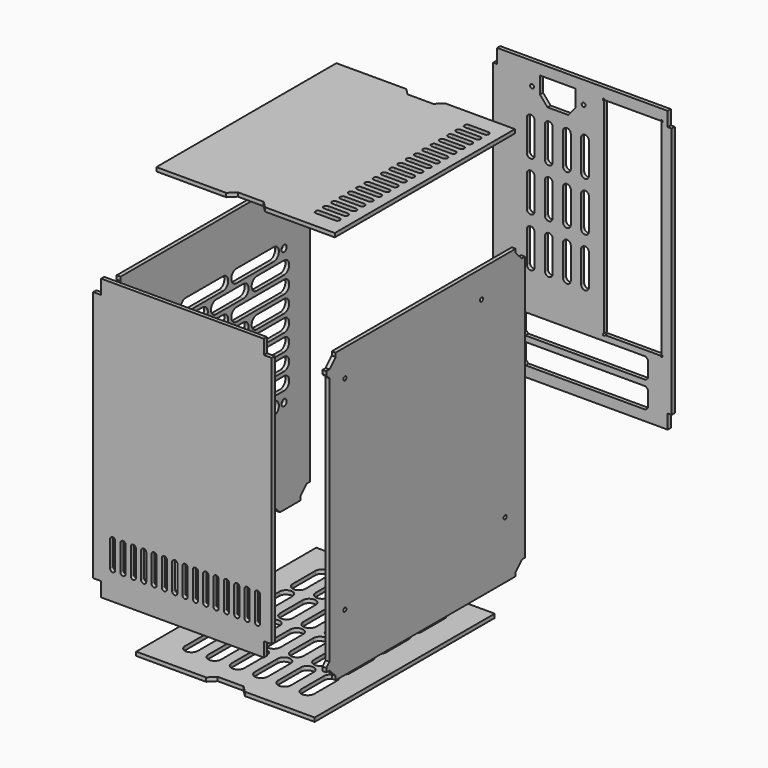
from build123d import *

# Parameters (mm, degrees)
F1_DEPTH  = 3
F4_DEPTH  = 3
F7_DEPTH  = 3
F9_R      = 1.5
F10_DEPTH = 25
F13_DEPTH = 3
F15_R     = 2.5
F16_DEPTH = 25
F19_DEPTH = 3
F22_DEPTH = 25
F25_DEPTH = 3
F29_DEPTH = 25
F31_DEPTH = 3
F33_W     = 97
F33_H     = 15.9
F34_R     = 1.5
F35_DEPTH = 25
F36_SIZE  = 2


# Not quite as in the source:
# - a feature names something its author has since deleted; it is built from what else it names


with BuildPart() as f1:
    # F0 (on Front) → F1 (new body)
    with BuildSketch(Plane.XZ):
        Polygon((53.4554532792, 111.99751333), (-72.3445467208, 111.99751333), (-72.3445467208, 100.89751333), (-78.4445467208, 100.89751333), (-78.4445467208, 3.49751333), (59.5554532792, 3.49751333), (59.5554532792, 100.89751333), (53.4554532792, 100.89751333), align=None)
    extrude(amount=F1_DEPTH)

    # F2: F1 across face


with BuildPart() as f1_1:
    add(f1.part)
    add(f1.part.mirror(Plane(origin=(-9.4445467208, -1.5, 3.49751333), x_dir=(1, 0, 0), z_dir=(0, 0, -1))))

    # F3 (on face) → F4 (cut)
    with BuildSketch(Plane.XZ.offset(3)):
        with BuildLine():
            ThreePointArc((-61.4445467208, -63.00248667), (-63.4445467208, -61.00248667), (-65.4445467208, -63.00248667))
            Line((-65.4445467208, -63.00248667), (-65.4445467208, -83.00248667))
            ThreePointArc((-65.4445467208, -83.00248667), (-63.4445467208, -85.00248667), (-61.4445467208, -83.00248667))
            Line((-61.4445467208, -83.00248667), (-61.4445467208, -63.00248667))
        make_face()
        with BuildLine():
            ThreePointArc((-53.4445467208, -63.00248667), (-55.4445467208, -61.00248667), (-57.4445467208, -63.00248667))
            Line((-57.4445467208, -63.00248667), (-57.4445467208, -83.00248667))
            ThreePointArc((-57.4445467208, -83.00248667), (-55.4445467208, -85.00248667), (-53.4445467208, -83.00248667))
            Line((-53.4445467208, -83.00248667), (-53.4445467208, -63.00248667))
        make_face()
        with BuildLine():
            ThreePointArc((-45.4445467208, -63.00248667), (-47.4445467208, -61.00248667), (-49.4445467208, -63.00248667))
            Line((-49.4445467208, -63.00248667), (-49.4445467208, -83.00248667))
            ThreePointArc((-49.4445467208, -83.00248667), (-47.4445467208, -85.00248667), (-45.4445467208, -83.00248667))
            Line((-45.4445467208, -83.00248667), (-45.4445467208, -63.00248667))
        make_face()
        with BuildLine():
            ThreePointArc((-37.4445467208, -63.00248667), (-39.4445467208, -61.00248667), (-41.4445467208, -63.00248667))
            Line((-41.4445467208, -63.00248667), (-41.4445467208, -83.00248667))
            ThreePointArc((-41.4445467208, -83.00248667), (-39.4445467208, -85.00248667), (-37.4445467208, -83.00248667))
            Line((-37.4445467208, -83.00248667), (-37.4445467208, -63.00248667))
        make_face()
        with BuildLine():
            ThreePointArc((-29.4445467208, -63.00248667), (-31.4445467208, -61.00248667), (-33.4445467208, -63.00248667))
            Line((-33.4445467208, -63.00248667), (-33.4445467208, -83.00248667))
            ThreePointArc((-33.4445467208, -83.00248667), (-31.4445467208, -85.00248667), (-29.4445467208, -83.00248667))
            Line((-29.4445467208, -83.00248667), (-29.4445467208, -63.00248667))
        make_face()
        with BuildLine():
            ThreePointArc((-21.4445467208, -63.00248667), (-23.4445467208, -61.00248667), (-25.4445467208, -63.00248667))
            Line((-25.4445467208, -63.00248667), (-25.4445467208, -83.00248667))
            ThreePointArc((-25.4445467208, -83.00248667), (-23.4445467208, -85.00248667), (-21.4445467208, -83.00248667))
            Line((-21.4445467208, -83.00248667), (-21.4445467208, -63.00248667))
        make_face()
        with BuildLine():
            ThreePointArc((-13.4445467208, -63.00248667), (-15.4445467208, -61.00248667), (-17.4445467208, -63.00248667))
            Line((-17.4445467208, -63.00248667), (-17.4445467208, -83.00248667))
            ThreePointArc((-17.4445467208, -83.00248667), (-15.4445467208, -85.00248667), (-13.4445467208, -83.00248667))
            Line((-13.4445467208, -83.00248667), (-13.4445467208, -63.00248667))
        make_face()
        with BuildLine():
            ThreePointArc((-5.4445467208, -63.00248667), (-7.4445467208, -61.00248667), (-9.4445467208, -63.00248667))
            Line((-9.4445467208, -63.00248667), (-9.4445467208, -83.00248667))
            ThreePointArc((-9.4445467208, -83.00248667), (-7.4445467208, -85.00248667), (-5.4445467208, -83.00248667))
            Line((-5.4445467208, -83.00248667), (-5.4445467208, -63.00248667))
        make_face()
        with BuildLine():
            ThreePointArc((2.5554532792, -63.00248667), (0.5554532792, -61.00248667), (-1.4445467208, -63.00248667))
            Line((-1.4445467208, -63.00248667), (-1.4445467208, -83.00248667))
            ThreePointArc((-1.4445467208, -83.00248667), (0.5554532792, -85.00248667), (2.5554532792, -83.00248667))
            Line((2.5554532792, -83.00248667), (2.5554532792, -63.00248667))
        make_face()
        with BuildLine():
            ThreePointArc((10.5554532792, -63.00248667), (8.5554532792, -61.00248667), (6.5554532792, -63.00248667))
            Line((6.5554532792, -63.00248667), (6.5554532792, -83.00248667))
            ThreePointArc((6.5554532792, -83.00248667), (8.5554532792, -85.00248667), (10.5554532792, -83.00248667))
            Line((10.5554532792, -83.00248667), (10.5554532792, -63.00248667))
        make_face()
        with BuildLine():
            ThreePointArc((18.5554532792, -63.00248667), (16.5554532792, -61.00248667), (14.5554532792, -63.00248667))
            Line((14.5554532792, -63.00248667), (14.5554532792, -83.00248667))
            ThreePointArc((14.5554532792, -83.00248667), (16.5554532792, -85.00248667), (18.5554532792, -83.00248667))
            Line((18.5554532792, -83.00248667), (18.5554532792, -63.00248667))
        make_face()
        with BuildLine():
            ThreePointArc((26.5554532792, -63.00248667), (24.5554532792, -61.00248667), (22.5554532792, -63.00248667))
            Line((22.5554532792, -63.00248667), (22.5554532792, -83.00248667))
            ThreePointArc((22.5554532792, -83.00248667), (24.5554532792, -85.00248667), (26.5554532792, -83.00248667))
            Line((26.5554532792, -83.00248667), (26.5554532792, -63.00248667))
        make_face()
        with BuildLine():
            ThreePointArc((34.5554532792, -63.00248667), (32.5554532792, -61.00248667), (30.5554532792, -63.00248667))
            Line((30.5554532792, -63.00248667), (30.5554532792, -83.00248667))
            ThreePointArc((30.5554532792, -83.00248667), (32.5554532792, -85.00248667), (34.5554532792, -83.00248667))
            Line((34.5554532792, -83.00248667), (34.5554532792, -63.00248667))
        make_face()
        with BuildLine():
            ThreePointArc((42.5554532792, -63.00248667), (40.5554532792, -61.00248667), (38.5554532792, -63.00248667))
            Line((38.5554532792, -63.00248667), (38.5554532792, -83.00248667))
            ThreePointArc((38.5554532792, -83.00248667), (40.5554532792, -85.00248667), (42.5554532792, -83.00248667))
            Line((42.5554532792, -83.00248667), (42.5554532792, -63.00248667))
        make_face()
        with BuildLine():
            ThreePointArc((50.5554532792, -63.00248667), (48.5554532792, -61.00248667), (46.5554532792, -63.00248667))
            Line((46.5554532792, -63.00248667), (46.5554532792, -83.00248667))
            ThreePointArc((46.5554532792, -83.00248667), (48.5554532792, -85.00248667), (50.5554532792, -83.00248667))
            Line((50.5554532792, -83.00248667), (50.5554532792, -63.00248667))
        make_face()
    extrude(amount=-F4_DEPTH, mode=Mode.SUBTRACT)


with BuildPart() as f7:
    # F6 (on offset) → F7 (new body)
    with BuildSketch(Plane.YZ.offset(80)):
        Polygon((203.4780200328, 98.9318754673), (29.4780200328, 98.9318754673), (29.4780200328, 95.9318754673), (23.4780200328, 89.9318754673), (20.4780200328, 89.9318754673), (20.4780200328, 86.9318754673), (23.4780200328, 83.9318754673), (23.4780200328, -12.5681245327), (209.4780200328, -12.5681245327), (209.4780200328, 83.9318754673), (212.4780200328, 86.9318754673), (212.4780200328, 89.9318754673), (209.4780200328, 89.9318754673), (203.4780200328, 95.9318754673), align=None)
        Polygon((212.4780200328, -12.5681245327), (212.4780200328, 86.9318754673), (209.4780200328, 83.9318754673), (209.4780200328, -12.5681245327), align=None)
    extrude(amount=F7_DEPTH)

    # F8: F7 across face


with BuildPart() as f7_1:
    add(f7.part)
    add(f7.part.mirror(Plane(origin=(81.5, 117.9780200328, -12.5681245327), x_dir=(1, 0, 0), z_dir=(0, 0, -1))))

    # F9 (on face) → F10 (cut)
    with BuildSketch(Plane.YZ.offset(83)):
        with Locations((38.3780200328, -79.6681245327)):
            Circle(F9_R)
        with Locations((38.3780200328, 77.7318754673)):
            Circle(F9_R)
        with Locations((170.4780200328, 77.7318754673)):
            Circle(F9_R)
        with Locations((193.2780200328, -79.6681245327)):
            Circle(F9_R)
    extrude(amount=-F10_DEPTH, mode=Mode.SUBTRACT)


with BuildPart() as f13:
    # F12 (on offset) → F13 (new body)
    with BuildSketch(Plane.YZ.offset(-96)):
        Polygon((215.6347262859, 85.4871258276), (215.6347262859, 88.4871258276), (41.6347262859, 88.4871258276), (41.6347262859, 85.4871258276), (35.6347262859, 79.4871258276), (32.6347262859, 79.4871258276), (32.6347262859, 76.4871258276), (35.6347262859, 73.4871258276), (35.6347262859, -23.0128741724), (224.6347262859, -23.0128741724), (224.6347262859, 79.4871258276), (221.6347262859, 79.4871258276), align=None)
    extrude(amount=F13_DEPTH)

    # F14: F13 across face


with BuildPart() as f13_1:
    add(f13.part)
    add(f13.part.mirror(Plane(origin=(-94.5, 130.1347262859, -23.0128741724), x_dir=(1, 0, 0), z_dir=(0, 0, -1))))

    # F15 (on face) → F16 (cut)
    with BuildSketch(Plane(origin=(-96, 0, 0), x_dir=(0, -1, 0), z_dir=(-1, 0, 0))):
        with Locations((-199.6347262859, 43.4871258276)):
            Circle(F15_R)
        with Locations((-94.6347262859, 43.4871258276)):
            Circle(F15_R)
        with BuildLine():
            ThreePointArc((-189.6347262859, 48.4871258276), (-194.6347262859, 43.4871258276), (-189.6347262859, 38.4871258276))
            Line((-189.6347262859, 38.4871258276), (-153.6347262859, 38.4871258276))
            ThreePointArc((-153.6347262859, 38.4871258276), (-148.6347262859, 43.4871258276), (-153.6347262859, 48.4871258276))
            Line((-153.6347262859, 48.4871258276), (-189.6347262859, 48.4871258276))
        make_face()
        with BuildLine():
            ThreePointArc((-140.6347262859, 48.4871258276), (-145.6347262859, 43.4871258276), (-140.6347262859, 38.4871258276))
            Line((-140.6347262859, 38.4871258276), (-104.6347262859, 38.4871258276))
            ThreePointArc((-104.6347262859, 38.4871258276), (-99.6347262859, 43.4871258276), (-104.6347262859, 48.4871258276))
            Line((-104.6347262859, 48.4871258276), (-140.6347262859, 48.4871258276))
        make_face()
        with BuildLine():
            ThreePointArc((-199.6347262859, 35.3621258276), (-204.6347262859, 30.3621258276), (-199.6347262859, 25.3621258276))
            Line((-199.6347262859, 25.3621258276), (-173.3013929526, 25.3621258276))
            ThreePointArc((-173.3013929526, 25.3621258276), (-168.3013929526, 30.3621258276), (-173.3013929526, 35.3621258276))
            Line((-173.3013929526, 35.3621258276), (-199.6347262859, 35.3621258276))
        make_face()
        with BuildLine():
            ThreePointArc((-160.3013929526, 35.3621258276), (-165.3013929526, 30.3621258276), (-160.3013929526, 25.3621258276))
            Line((-160.3013929526, 25.3621258276), (-133.9680596193, 25.3621258276))
            ThreePointArc((-133.9680596193, 25.3621258276), (-128.9680596193, 30.3621258276), (-133.9680596193, 35.3621258276))
            Line((-133.9680596193, 35.3621258276), (-160.3013929526, 35.3621258276))
        make_face()
        with BuildLine():
            ThreePointArc((-120.9680596193, 35.3621258276), (-125.9680596193, 30.3621258276), (-120.9680596193, 25.3621258276))
            Line((-120.9680596193, 25.3621258276), (-94.6347262859, 25.3621258276))
            ThreePointArc((-94.6347262859, 25.3621258276), (-89.6347262859, 30.3621258276), (-94.6347262859, 35.3621258276))
            Line((-94.6347262859, 35.3621258276), (-120.9680596193, 35.3621258276))
        make_face()
        with BuildLine():
            ThreePointArc((-199.6347262859, 22.2371258276), (-204.6347262859, 17.2371258276), (-199.6347262859, 12.2371258276))
            Line((-199.6347262859, 12.2371258276), (-153.6347262859, 12.2371258276))
            ThreePointArc((-153.6347262859, 12.2371258276), (-148.6347262859, 17.2371258276), (-153.6347262859, 22.2371258276))
            Line((-153.6347262859, 22.2371258276), (-199.6347262859, 22.2371258276))
        make_face()
        with BuildLine():
            ThreePointArc((-140.6347262859, 22.2371258276), (-145.6347262859, 17.2371258276), (-140.6347262859, 12.2371258276))
            Line((-140.6347262859, 12.2371258276), (-94.6347262859, 12.2371258276))
            ThreePointArc((-94.6347262859, 12.2371258276), (-89.6347262859, 17.2371258276), (-94.6347262859, 22.2371258276))
            Line((-94.6347262859, 22.2371258276), (-140.6347262859, 22.2371258276))
        make_face()
        with BuildLine():
            ThreePointArc((-199.6347262859, 9.1121258276), (-204.6347262859, 4.1121258276), (-199.6347262859, -0.8878741724))
            Line((-199.6347262859, -0.8878741724), (-173.3013929526, -0.8878741724))
            ThreePointArc((-173.3013929526, -0.8878741724), (-168.3013929526, 4.1121258276), (-173.3013929526, 9.1121258276))
            Line((-173.3013929526, 9.1121258276), (-199.6347262859, 9.1121258276))
        make_face()
        with BuildLine():
            ThreePointArc((-160.3013929526, 9.1121258276), (-165.3013929526, 4.1121258276), (-160.3013929526, -0.8878741724))
            Line((-160.3013929526, -0.8878741724), (-133.9680596193, -0.8878741724))
            ThreePointArc((-133.9680596193, -0.8878741724), (-128.9680596193, 4.1121258276), (-133.9680596193, 9.1121258276))
            Line((-133.9680596193, 9.1121258276), (-160.3013929526, 9.1121258276))
        make_face()
        with BuildLine():
            ThreePointArc((-120.9680596193, 9.1121258276), (-125.9680596193, 4.1121258276), (-120.9680596193, -0.8878741724))
            Line((-120.9680596193, -0.8878741724), (-94.6347262859, -0.8878741724))
            ThreePointArc((-94.6347262859, -0.8878741724), (-89.6347262859, 4.1121258276), (-94.6347262859, 9.1121258276))
            Line((-94.6347262859, 9.1121258276), (-120.9680596193, 9.1121258276))
        make_face()
        with BuildLine():
            ThreePointArc((-199.6347262859, -4.0128741724), (-204.6347262859, -9.0128741724), (-199.6347262859, -14.0128741724))
            Line((-199.6347262859, -14.0128741724), (-153.6347262859, -14.0128741724))
            ThreePointArc((-153.6347262859, -14.0128741724), (-148.6347262859, -9.0128741724), (-153.6347262859, -4.0128741724))
            Line((-153.6347262859, -4.0128741724), (-199.6347262859, -4.0128741724))
        make_face()
        with BuildLine():
            ThreePointArc((-140.6347262859, -4.0128741724), (-145.6347262859, -9.0128741724), (-140.6347262859, -14.0128741724))
            Line((-140.6347262859, -14.0128741724), (-94.6347262859, -14.0128741724))
            ThreePointArc((-94.6347262859, -14.0128741724), (-89.6347262859, -9.0128741724), (-94.6347262859, -4.0128741724))
            Line((-94.6347262859, -4.0128741724), (-140.6347262859, -4.0128741724))
        make_face()
        with BuildLine():
            ThreePointArc((-199.6347262859, -17.1378741724), (-204.6347262859, -22.1378741724), (-199.6347262859, -27.1378741724))
            Line((-199.6347262859, -27.1378741724), (-173.3013929526, -27.1378741724))
            ThreePointArc((-173.3013929526, -27.1378741724), (-168.3013929526, -22.1378741724), (-173.3013929526, -17.1378741724))
            Line((-173.3013929526, -17.1378741724), (-199.6347262859, -17.1378741724))
        make_face()
        with BuildLine():
            ThreePointArc((-160.3013929526, -17.1378741724), (-165.3013929526, -22.1378741724), (-160.3013929526, -27.1378741724))
            Line((-160.3013929526, -27.1378741724), (-133.9680596193, -27.1378741724))
            ThreePointArc((-133.9680596193, -27.1378741724), (-128.9680596193, -22.1378741724), (-133.9680596193, -17.1378741724))
            Line((-133.9680596193, -17.1378741724), (-160.3013929526, -17.1378741724))
        make_face()
        with BuildLine():
            ThreePointArc((-120.9680596193, -17.1378741724), (-125.9680596193, -22.1378741724), (-120.9680596193, -27.1378741724))
            Line((-120.9680596193, -27.1378741724), (-94.6347262859, -27.1378741724))
            ThreePointArc((-94.6347262859, -27.1378741724), (-89.6347262859, -22.1378741724), (-94.6347262859, -17.1378741724))
            Line((-94.6347262859, -17.1378741724), (-120.9680596193, -17.1378741724))
        make_face()
        with BuildLine():
            ThreePointArc((-199.6347262859, -30.2628741724), (-204.6347262859, -35.2628741724), (-199.6347262859, -40.2628741724))
            Line((-199.6347262859, -40.2628741724), (-153.6347262859, -40.2628741724))
            ThreePointArc((-153.6347262859, -40.2628741724), (-148.6347262859, -35.2628741724), (-153.6347262859, -30.2628741724))
            Line((-153.6347262859, -30.2628741724), (-199.6347262859, -30.2628741724))
        make_face()
        with BuildLine():
            ThreePointArc((-140.6347262859, -30.2628741724), (-145.6347262859, -35.2628741724), (-140.6347262859, -40.2628741724))
            Line((-140.6347262859, -40.2628741724), (-94.6347262859, -40.2628741724))
            ThreePointArc((-94.6347262859, -40.2628741724), (-89.6347262859, -35.2628741724), (-94.6347262859, -30.2628741724))
            Line((-94.6347262859, -30.2628741724), (-140.6347262859, -30.2628741724))
        make_face()
        with BuildLine():
            ThreePointArc((-199.6347262859, -43.3878741724), (-204.6347262859, -48.3878741724), (-199.6347262859, -53.3878741724))
            Line((-199.6347262859, -53.3878741724), (-173.3013929526, -53.3878741724))
            ThreePointArc((-173.3013929526, -53.3878741724), (-168.3013929526, -48.3878741724), (-173.3013929526, -43.3878741724))
            Line((-173.3013929526, -43.3878741724), (-199.6347262859, -43.3878741724))
        make_face()
        with BuildLine():
            ThreePointArc((-160.3013929526, -43.3878741724), (-165.3013929526, -48.3878741724), (-160.3013929526, -53.3878741724))
            Line((-160.3013929526, -53.3878741724), (-133.9680596193, -53.3878741724))
            ThreePointArc((-133.9680596193, -53.3878741724), (-128.9680596193, -48.3878741724), (-133.9680596193, -43.3878741724))
            Line((-133.9680596193, -43.3878741724), (-160.3013929526, -43.3878741724))
        make_face()
        with BuildLine():
            ThreePointArc((-120.9680596193, -43.3878741724), (-125.9680596193, -48.3878741724), (-120.9680596193, -53.3878741724))
            Line((-120.9680596193, -53.3878741724), (-94.6347262859, -53.3878741724))
            ThreePointArc((-94.6347262859, -53.3878741724), (-89.6347262859, -48.3878741724), (-94.6347262859, -43.3878741724))
            Line((-94.6347262859, -43.3878741724), (-120.9680596193, -43.3878741724))
        make_face()
        with BuildLine():
            ThreePointArc((-189.6347262859, -56.5128741724), (-194.6347262859, -61.5128741724), (-189.6347262859, -66.5128741724))
            Line((-189.6347262859, -66.5128741724), (-153.6347262859, -66.5128741724))
            ThreePointArc((-153.6347262859, -66.5128741724), (-148.6347262859, -61.5128741724), (-153.6347262859, -56.5128741724))
            Line((-153.6347262859, -56.5128741724), (-189.6347262859, -56.5128741724))
        make_face()
        with BuildLine():
            ThreePointArc((-140.6347262859, -56.5128741724), (-145.6347262859, -61.5128741724), (-140.6347262859, -66.5128741724))
            Line((-140.6347262859, -66.5128741724), (-104.6347262859, -66.5128741724))
            ThreePointArc((-104.6347262859, -66.5128741724), (-99.6347262859, -61.5128741724), (-104.6347262859, -56.5128741724))
            Line((-104.6347262859, -56.5128741724), (-140.6347262859, -56.5128741724))
        make_face()
        with Locations((-199.6347262859, -61.5128741724)):
            Circle(F15_R)
        with Locations((-94.6347262859, -61.5128741724)):
            Circle(F15_R)
        Polygon((-187.6347262859, -126.5128741724), (-195.6347262859, -134.5128741724), (-61.6347262859, -134.5128741724), (-69.6347262859, -126.5128741724), align=None)
    extrude(amount=-F16_DEPTH, mode=Mode.SUBTRACT)


with BuildPart() as f19:
    # F18 (on offset) → F19 (new body)
    with BuildSketch(Plane.XY.offset(155)):
        Polygon((55.7591726665, 149.7526661158), (-82.2408273335, 149.7526661158), (-82.2408273335, 62.7526661158), (-28.2408273335, 62.7526661158), (-23.2408273335, 67.7526661158), (-13.2408273335, 67.7526661158), (-3.2408273335, 67.7526661158), (1.7591726665, 62.7526661158), (55.7591726665, 62.7526661158), align=None)
    extrude(amount=F19_DEPTH)

    # F20: F19 across face


with BuildPart() as f19_1:
    add(f19.part)
    add(f19.part.mirror(Plane(origin=(-13.2408273335, 149.7526661158, 156.5), x_dir=(-1, 0, 0), z_dir=(0, 1, 0))))

    # F21 (on face) → F22 (cut)
    with BuildSketch(Plane.XY.offset(158)):
        with BuildLine():
            ThreePointArc((30.7591726665, 79.7526661158), (28.7591726665, 77.7526661158), (30.7591726665, 75.7526661158))
            Line((30.7591726665, 75.7526661158), (45.7591726665, 75.7526661158))
            ThreePointArc((45.7591726665, 75.7526661158), (47.7591726665, 77.7526661158), (45.7591726665, 79.7526661158))
            Line((45.7591726665, 79.7526661158), (30.7591726665, 79.7526661158))
        make_face()
        with BuildLine():
            ThreePointArc((30.7591726665, 87.7526661158), (28.7591726665, 85.7526661158), (30.7591726665, 83.7526661158))
            Line((30.7591726665, 83.7526661158), (45.7591726665, 83.7526661158))
            ThreePointArc((45.7591726665, 83.7526661158), (47.7591726665, 85.7526661158), (45.7591726665, 87.7526661158))
            Line((45.7591726665, 87.7526661158), (30.7591726665, 87.7526661158))
        make_face()
        with BuildLine():
            ThreePointArc((30.7591726665, 95.7526661158), (28.7591726665, 93.7526661158), (30.7591726665, 91.7526661158))
            Line((30.7591726665, 91.7526661158), (45.7591726665, 91.7526661158))
            ThreePointArc((45.7591726665, 91.7526661158), (47.7591726665, 93.7526661158), (45.7591726665, 95.7526661158))
            Line((45.7591726665, 95.7526661158), (30.7591726665, 95.7526661158))
        make_face()
        with BuildLine():
            ThreePointArc((30.7591726665, 103.7526661158), (28.7591726665, 101.7526661158), (30.7591726665, 99.7526661158))
            Line((30.7591726665, 99.7526661158), (45.7591726665, 99.7526661158))
            ThreePointArc((45.7591726665, 99.7526661158), (47.7591726665, 101.7526661158), (45.7591726665, 103.7526661158))
            Line((45.7591726665, 103.7526661158), (30.7591726665, 103.7526661158))
        make_face()
        with BuildLine():
            ThreePointArc((30.7591726665, 111.7526661158), (28.7591726665, 109.7526661158), (30.7591726665, 107.7526661158))
            Line((30.7591726665, 107.7526661158), (45.7591726665, 107.7526661158))
            ThreePointArc((45.7591726665, 107.7526661158), (47.7591726665, 109.7526661158), (45.7591726665, 111.7526661158))
            Line((45.7591726665, 111.7526661158), (30.7591726665, 111.7526661158))
        make_face()
        with BuildLine():
            ThreePointArc((30.7591726665, 119.7526661158), (28.7591726665, 117.7526661158), (30.7591726665, 115.7526661158))
            Line((30.7591726665, 115.7526661158), (45.7591726665, 115.7526661158))
            ThreePointArc((45.7591726665, 115.7526661158), (47.7591726665, 117.7526661158), (45.7591726665, 119.7526661158))
            Line((45.7591726665, 119.7526661158), (30.7591726665, 119.7526661158))
        make_face()
        with BuildLine():
            ThreePointArc((30.7591726665, 127.7526661158), (28.7591726665, 125.7526661158), (30.7591726665, 123.7526661158))
            Line((30.7591726665, 123.7526661158), (45.7591726665, 123.7526661158))
            ThreePointArc((45.7591726665, 123.7526661158), (47.7591726665, 125.7526661158), (45.7591726665, 127.7526661158))
            Line((45.7591726665, 127.7526661158), (30.7591726665, 127.7526661158))
        make_face()
        with BuildLine():
            ThreePointArc((30.7591726665, 135.7526661158), (28.7591726665, 133.7526661158), (30.7591726665, 131.7526661158))
            Line((30.7591726665, 131.7526661158), (45.7591726665, 131.7526661158))
            ThreePointArc((45.7591726665, 131.7526661158), (47.7591726665, 133.7526661158), (45.7591726665, 135.7526661158))
            Line((45.7591726665, 135.7526661158), (30.7591726665, 135.7526661158))
        make_face()
        with BuildLine():
            ThreePointArc((30.7591726665, 143.7526661158), (28.7591726665, 141.7526661158), (30.7591726665, 139.7526661158))
            Line((30.7591726665, 139.7526661158), (45.7591726665, 139.7526661158))
            ThreePointArc((45.7591726665, 139.7526661158), (47.7591726665, 141.7526661158), (45.7591726665, 143.7526661158))
            Line((45.7591726665, 143.7526661158), (30.7591726665, 143.7526661158))
        make_face()
        with BuildLine():
            ThreePointArc((30.7591726665, 151.7526661158), (28.7591726665, 149.7526661158), (30.7591726665, 147.7526661158))
            Line((30.7591726665, 147.7526661158), (45.7591726665, 147.7526661158))
            ThreePointArc((45.7591726665, 147.7526661158), (47.7591726665, 149.7526661158), (45.7591726665, 151.7526661158))
            Line((45.7591726665, 151.7526661158), (30.7591726665, 151.7526661158))
        make_face()
        with BuildLine():
            ThreePointArc((30.7591726665, 159.7526661158), (28.7591726665, 157.7526661158), (30.7591726665, 155.7526661158))
            Line((30.7591726665, 155.7526661158), (45.7591726665, 155.7526661158))
            ThreePointArc((45.7591726665, 155.7526661158), (47.7591726665, 157.7526661158), (45.7591726665, 159.7526661158))
            Line((45.7591726665, 159.7526661158), (30.7591726665, 159.7526661158))
        make_face()
        with BuildLine():
            ThreePointArc((30.7591726665, 167.7526661158), (28.7591726665, 165.7526661158), (30.7591726665, 163.7526661158))
            Line((30.7591726665, 163.7526661158), (45.7591726665, 163.7526661158))
            ThreePointArc((45.7591726665, 163.7526661158), (47.7591726665, 165.7526661158), (45.7591726665, 167.7526661158))
            Line((45.7591726665, 167.7526661158), (30.7591726665, 167.7526661158))
        make_face()
        with BuildLine():
            ThreePointArc((30.7591726665, 175.7526661158), (28.7591726665, 173.7526661158), (30.7591726665, 171.7526661158))
            Line((30.7591726665, 171.7526661158), (45.7591726665, 171.7526661158))
            ThreePointArc((45.7591726665, 171.7526661158), (47.7591726665, 173.7526661158), (45.7591726665, 175.7526661158))
            Line((45.7591726665, 175.7526661158), (30.7591726665, 175.7526661158))
        make_face()
        with BuildLine():
            ThreePointArc((30.7591726665, 183.7526661158), (28.7591726665, 181.7526661158), (30.7591726665, 179.7526661158))
            Line((30.7591726665, 179.7526661158), (45.7591726665, 179.7526661158))
            ThreePointArc((45.7591726665, 179.7526661158), (47.7591726665, 181.7526661158), (45.7591726665, 183.7526661158))
            Line((45.7591726665, 183.7526661158), (30.7591726665, 183.7526661158))
        make_face()
        with BuildLine():
            ThreePointArc((30.7591726665, 191.7526661158), (28.7591726665, 189.7526661158), (30.7591726665, 187.7526661158))
            Line((30.7591726665, 187.7526661158), (45.7591726665, 187.7526661158))
            ThreePointArc((45.7591726665, 187.7526661158), (47.7591726665, 189.7526661158), (45.7591726665, 191.7526661158))
            Line((45.7591726665, 191.7526661158), (30.7591726665, 191.7526661158))
        make_face()
        with BuildLine():
            ThreePointArc((30.7591726665, 199.7526661158), (28.7591726665, 197.7526661158), (30.7591726665, 195.7526661158))
            Line((30.7591726665, 195.7526661158), (45.7591726665, 195.7526661158))
            ThreePointArc((45.7591726665, 195.7526661158), (47.7591726665, 197.7526661158), (45.7591726665, 199.7526661158))
            Line((45.7591726665, 199.7526661158), (30.7591726665, 199.7526661158))
        make_face()
        with BuildLine():
            ThreePointArc((30.7591726665, 207.7526661158), (28.7591726665, 205.7526661158), (30.7591726665, 203.7526661158))
            Line((30.7591726665, 203.7526661158), (45.7591726665, 203.7526661158))
            ThreePointArc((45.7591726665, 203.7526661158), (47.7591726665, 205.7526661158), (45.7591726665, 207.7526661158))
            Line((45.7591726665, 207.7526661158), (30.7591726665, 207.7526661158))
        make_face()
        with BuildLine():
            ThreePointArc((30.7591726665, 215.7526661158), (28.7591726665, 213.7526661158), (30.7591726665, 211.7526661158))
            Line((30.7591726665, 211.7526661158), (45.7591726665, 211.7526661158))
            ThreePointArc((45.7591726665, 211.7526661158), (47.7591726665, 213.7526661158), (45.7591726665, 215.7526661158))
            Line((45.7591726665, 215.7526661158), (30.7591726665, 215.7526661158))
        make_face()
        with BuildLine():
            ThreePointArc((30.7591726665, 223.7526661158), (28.7591726665, 221.7526661158), (30.7591726665, 219.7526661158))
            Line((30.7591726665, 219.7526661158), (45.7591726665, 219.7526661158))
            ThreePointArc((45.7591726665, 219.7526661158), (47.7591726665, 221.7526661158), (45.7591726665, 223.7526661158))
            Line((45.7591726665, 223.7526661158), (30.7591726665, 223.7526661158))
        make_face()
    extrude(amount=-F22_DEPTH, mode=Mode.SUBTRACT)


with BuildPart() as f25:
    # F24 (on offset) → F25 (new body)
    with BuildSketch(Plane.XY.offset(-153)):
        Polygon((-65.5607343912, 109.4242391139), (-65.5607343912, 22.4242391139), (-11.5607343912, 22.4242391139), (-6.5607343912, 27.4242391139), (3.4392656088, 27.4242391139), (13.4392656088, 27.4242391139), (18.4392656088, 22.4242391139), (72.4392656088, 22.4242391139), (72.4392656088, 109.4242391139), align=None)
    extrude(amount=F25_DEPTH)

    # F26: F25 across face


with BuildPart() as f25_1:
    add(f25.part)
    add(f25.part.mirror(Plane(origin=(3.4392656088, 109.4242391139, -151.5), x_dir=(-1, 0, 0), z_dir=(0, 1, 0))))

    # F28 (on face) → F29 (cut)
    with BuildSketch(Plane(origin=(0, 0, -153), x_dir=(1, 0, 0), z_dir=(0, 0, -1))):
        with BuildLine():
            ThreePointArc((-47.0607343912, -172.4242391139), (-42.0607343912, -177.4242391139), (-37.0607343912, -172.4242391139))
            Line((-37.0607343912, -172.4242391139), (-37.0607343912, -150.4242391139))
            ThreePointArc((-37.0607343912, -150.4242391139), (-42.0607343912, -145.4242391139), (-47.0607343912, -150.4242391139))
            Line((-47.0607343912, -150.4242391139), (-47.0607343912, -172.4242391139))
        make_face()
        with BuildLine():
            ThreePointArc((-47.0607343912, -137.7575724473), (-42.0607343912, -142.7575724473), (-37.0607343912, -137.7575724473))
            Line((-37.0607343912, -137.7575724473), (-37.0607343912, -115.7575724473))
            ThreePointArc((-37.0607343912, -115.7575724473), (-42.0607343912, -110.7575724473), (-47.0607343912, -115.7575724473))
            Line((-47.0607343912, -115.7575724473), (-47.0607343912, -137.7575724473))
        make_face()
        with BuildLine():
            ThreePointArc((-47.0607343912, -103.0909057806), (-42.0607343912, -108.0909057806), (-37.0607343912, -103.0909057806))
            Line((-37.0607343912, -103.0909057806), (-37.0607343912, -81.0909057806))
            ThreePointArc((-37.0607343912, -81.0909057806), (-42.0607343912, -76.0909057806), (-47.0607343912, -81.0909057806))
            Line((-47.0607343912, -81.0909057806), (-47.0607343912, -103.0909057806))
        make_face()
        with BuildLine():
            ThreePointArc((-47.0607343912, -68.4242391139), (-42.0607343912, -73.4242391139), (-37.0607343912, -68.4242391139))
            Line((-37.0607343912, -68.4242391139), (-37.0607343912, -46.4242391139))
            ThreePointArc((-37.0607343912, -46.4242391139), (-42.0607343912, -41.4242391139), (-47.0607343912, -46.4242391139))
            Line((-47.0607343912, -46.4242391139), (-47.0607343912, -68.4242391139))
        make_face()
        with BuildLine():
            ThreePointArc((-29.0607343912, -172.4242391139), (-24.0607343912, -177.4242391139), (-19.0607343912, -172.4242391139))
            Line((-19.0607343912, -172.4242391139), (-19.0607343912, -150.4242391139))
            ThreePointArc((-19.0607343912, -150.4242391139), (-24.0607343912, -145.4242391139), (-29.0607343912, -150.4242391139))
            Line((-29.0607343912, -150.4242391139), (-29.0607343912, -172.4242391139))
        make_face()
        with BuildLine():
            ThreePointArc((-29.0607343912, -137.7575724473), (-24.0607343912, -142.7575724473), (-19.0607343912, -137.7575724473))
            Line((-19.0607343912, -137.7575724473), (-19.0607343912, -115.7575724473))
            ThreePointArc((-19.0607343912, -115.7575724473), (-24.0607343912, -110.7575724473), (-29.0607343912, -115.7575724473))
            Line((-29.0607343912, -115.7575724473), (-29.0607343912, -137.7575724473))
        make_face()
        with BuildLine():
            ThreePointArc((-29.0607343912, -103.0909057806), (-24.0607343912, -108.0909057806), (-19.0607343912, -103.0909057806))
            Line((-19.0607343912, -103.0909057806), (-19.0607343912, -81.0909057806))
            ThreePointArc((-19.0607343912, -81.0909057806), (-24.0607343912, -76.0909057806), (-29.0607343912, -81.0909057806))
            Line((-29.0607343912, -81.0909057806), (-29.0607343912, -103.0909057806))
        make_face()
        with BuildLine():
            ThreePointArc((-29.0607343912, -68.4242391139), (-24.0607343912, -73.4242391139), (-19.0607343912, -68.4242391139))
            Line((-19.0607343912, -68.4242391139), (-19.0607343912, -46.4242391139))
            ThreePointArc((-19.0607343912, -46.4242391139), (-24.0607343912, -41.4242391139), (-29.0607343912, -46.4242391139))
            Line((-29.0607343912, -46.4242391139), (-29.0607343912, -68.4242391139))
        make_face()
        with BuildLine():
            ThreePointArc((-11.0607343912, -172.4242391139), (-6.0607343912, -177.4242391139), (-1.0607343912, -172.4242391139))
            Line((-1.0607343912, -172.4242391139), (-1.0607343912, -150.4242391139))
            ThreePointArc((-1.0607343912, -150.4242391139), (-6.0607343912, -145.4242391139), (-11.0607343912, -150.4242391139))
            Line((-11.0607343912, -150.4242391139), (-11.0607343912, -172.4242391139))
        make_face()
        with BuildLine():
            ThreePointArc((-11.0607343912, -137.7575724473), (-6.0607343912, -142.7575724473), (-1.0607343912, -137.7575724473))
            Line((-1.0607343912, -137.7575724473), (-1.0607343912, -115.7575724473))
            ThreePointArc((-1.0607343912, -115.7575724473), (-6.0607343912, -110.7575724473), (-11.0607343912, -115.7575724473))
            Line((-11.0607343912, -115.7575724473), (-11.0607343912, -137.7575724473))
        make_face()
        with BuildLine():
            ThreePointArc((-11.0607343912, -103.0909057806), (-6.0607343912, -108.0909057806), (-1.0607343912, -103.0909057806))
            Line((-1.0607343912, -103.0909057806), (-1.0607343912, -81.0909057806))
            ThreePointArc((-1.0607343912, -81.0909057806), (-6.0607343912, -76.0909057806), (-11.0607343912, -81.0909057806))
            Line((-11.0607343912, -81.0909057806), (-11.0607343912, -103.0909057806))
        make_face()
        with BuildLine():
            ThreePointArc((-11.0607343912, -68.4242391139), (-6.0607343912, -73.4242391139), (-1.0607343912, -68.4242391139))
            Line((-1.0607343912, -68.4242391139), (-1.0607343912, -46.4242391139))
            ThreePointArc((-1.0607343912, -46.4242391139), (-6.0607343912, -41.4242391139), (-11.0607343912, -46.4242391139))
            Line((-11.0607343912, -46.4242391139), (-11.0607343912, -68.4242391139))
        make_face()
        with BuildLine():
            ThreePointArc((6.9392656088, -172.4242391139), (11.9392656088, -177.4242391139), (16.9392656088, -172.4242391139))
            Line((16.9392656088, -172.4242391139), (16.9392656088, -150.4242391139))
            ThreePointArc((16.9392656088, -150.4242391139), (11.9392656088, -145.4242391139), (6.9392656088, -150.4242391139))
            Line((6.9392656088, -150.4242391139), (6.9392656088, -172.4242391139))
        make_face()
        with BuildLine():
            ThreePointArc((6.9392656088, -137.7575724473), (11.9392656088, -142.7575724473), (16.9392656088, -137.7575724473))
            Line((16.9392656088, -137.7575724473), (16.9392656088, -115.7575724473))
            ThreePointArc((16.9392656088, -115.7575724473), (11.9392656088, -110.7575724473), (6.9392656088, -115.7575724473))
            Line((6.9392656088, -115.7575724473), (6.9392656088, -137.7575724473))
        make_face()
        with BuildLine():
            ThreePointArc((6.9392656088, -103.0909057806), (11.9392656088, -108.0909057806), (16.9392656088, -103.0909057806))
            Line((16.9392656088, -103.0909057806), (16.9392656088, -81.0909057806))
            ThreePointArc((16.9392656088, -81.0909057806), (11.9392656088, -76.0909057806), (6.9392656088, -81.0909057806))
            Line((6.9392656088, -81.0909057806), (6.9392656088, -103.0909057806))
        make_face()
        with BuildLine():
            ThreePointArc((6.9392656088, -68.4242391139), (11.9392656088, -73.4242391139), (16.9392656088, -68.4242391139))
            Line((16.9392656088, -68.4242391139), (16.9392656088, -46.4242391139))
            ThreePointArc((16.9392656088, -46.4242391139), (11.9392656088, -41.4242391139), (6.9392656088, -46.4242391139))
            Line((6.9392656088, -46.4242391139), (6.9392656088, -68.4242391139))
        make_face()
        with BuildLine():
            ThreePointArc((24.9392656088, -172.4242391139), (29.9392656088, -177.4242391139), (34.9392656088, -172.4242391139))
            Line((34.9392656088, -172.4242391139), (34.9392656088, -150.4242391139))
            ThreePointArc((34.9392656088, -150.4242391139), (29.9392656088, -145.4242391139), (24.9392656088, -150.4242391139))
            Line((24.9392656088, -150.4242391139), (24.9392656088, -172.4242391139))
        make_face()
        with BuildLine():
            ThreePointArc((24.9392656088, -137.7575724473), (29.9392656088, -142.7575724473), (34.9392656088, -137.7575724473))
            Line((34.9392656088, -137.7575724473), (34.9392656088, -115.7575724473))
            ThreePointArc((34.9392656088, -115.7575724473), (29.9392656088, -110.7575724473), (24.9392656088, -115.7575724473))
            Line((24.9392656088, -115.7575724473), (24.9392656088, -137.7575724473))
        make_face()
        with BuildLine():
            ThreePointArc((24.9392656088, -103.0909057806), (29.9392656088, -108.0909057806), (34.9392656088, -103.0909057806))
            Line((34.9392656088, -103.0909057806), (34.9392656088, -81.0909057806))
            ThreePointArc((34.9392656088, -81.0909057806), (29.9392656088, -76.0909057806), (24.9392656088, -81.0909057806))
            Line((24.9392656088, -81.0909057806), (24.9392656088, -103.0909057806))
        make_face()
        with BuildLine():
            ThreePointArc((24.9392656088, -68.4242391139), (29.9392656088, -73.4242391139), (34.9392656088, -68.4242391139))
            Line((34.9392656088, -68.4242391139), (34.9392656088, -46.4242391139))
            ThreePointArc((34.9392656088, -46.4242391139), (29.9392656088, -41.4242391139), (24.9392656088, -46.4242391139))
            Line((24.9392656088, -46.4242391139), (24.9392656088, -68.4242391139))
        make_face()
        with BuildLine():
            ThreePointArc((42.9392656088, -172.4242391139), (47.9392656088, -177.4242391139), (52.9392656088, -172.4242391139))
            Line((52.9392656088, -172.4242391139), (52.9392656088, -150.4242391139))
            ThreePointArc((52.9392656088, -150.4242391139), (47.9392656088, -145.4242391139), (42.9392656088, -150.4242391139))
            Line((42.9392656088, -150.4242391139), (42.9392656088, -172.4242391139))
        make_face()
        with BuildLine():
            ThreePointArc((42.9392656088, -137.7575724473), (47.9392656088, -142.7575724473), (52.9392656088, -137.7575724473))
            Line((52.9392656088, -137.7575724473), (52.9392656088, -115.7575724473))
            ThreePointArc((52.9392656088, -115.7575724473), (47.9392656088, -110.7575724473), (42.9392656088, -115.7575724473))
            Line((42.9392656088, -115.7575724473), (42.9392656088, -137.7575724473))
        make_face()
        with BuildLine():
            ThreePointArc((42.9392656088, -103.0909057806), (47.9392656088, -108.0909057806), (52.9392656088, -103.0909057806))
            Line((52.9392656088, -103.0909057806), (52.9392656088, -81.0909057806))
            ThreePointArc((52.9392656088, -81.0909057806), (47.9392656088, -76.0909057806), (42.9392656088, -81.0909057806))
            Line((42.9392656088, -81.0909057806), (42.9392656088, -103.0909057806))
        make_face()
        with BuildLine():
            ThreePointArc((42.9392656088, -68.4242391139), (47.9392656088, -73.4242391139), (52.9392656088, -68.4242391139))
            Line((52.9392656088, -68.4242391139), (52.9392656088, -46.4242391139))
            ThreePointArc((52.9392656088, -46.4242391139), (47.9392656088, -41.4242391139), (42.9392656088, -46.4242391139))
            Line((42.9392656088, -46.4242391139), (42.9392656088, -68.4242391139))
        make_face()
    extrude(amount=-F29_DEPTH, mode=Mode.SUBTRACT)


with BuildPart() as f31:
    # F30 (on offset) → F31 (new body)
    with BuildSketch(Plane.XZ.offset(-376)):
        Polygon((64.95, 117.9973174244), (-66.95, 117.9973174244), (-66.95, 106.9473174244), (-70, 106.9473174244), (-70, 9.4973174244), (68, 9.4973174244), (68, 106.9473174244), (64.95, 106.9473174244), align=None)
    extrude(amount=F31_DEPTH)

    # F32: F31 across face


with BuildPart() as f31_1:
    add(f31.part)
    add(f31.part.mirror(Plane(origin=(-1, 374.5, 9.4973174244), x_dir=(1, 0, 0), z_dir=(0, 0, -1))))

    # F33 (on face) + F34 (on face) → F35 (cut)
    with BuildSketch(Plane(origin=(0, 376, 0), x_dir=(-1, 0, 0), z_dir=(0, 1, 0))):
        with Locations((-1.4, -62.7026825756)):
            Rectangle(F33_W, F33_H)
        with Locations((-1.4, -83.0026825756)):
            Rectangle(F33_W, F33_H)
        Polygon((64, -37.3226825756), (51, -50.3226825756), (51, -90.9526825756), (54, -90.9526825756), (57, -87.9526825756), (66.95, -87.9526825756), (70, -87.9526825756), (70, -37.3226825756), align=None)
        Polygon((-15.6, 108.7473174244), (-15.6, 109.4973174244), (-16.35, 109.4973174244), (-59.55, 109.4973174244), (-60.3, 109.4973174244), (-60.3, 108.7473174244), (-60.3, -49.6526825756), (-60.3, -50.4026825756), (-59.55, -50.4026825756), (-16.35, -50.4026825756), (-15.6, -50.4026825756), (-15.6, -49.6526825756), align=None)
        with BuildLine():
            Line((-16.35, 109.4973174244), (-15.6, 109.4973174244))
            Line((-15.6, 109.4973174244), (-15.6, 108.7473174244))
            ThreePointArc((-15.6, 108.7473174244), (-15.0696699141, 110.0276475103), (-16.35, 109.4973174244))
        make_face()
        with BuildLine():
            Line((-60.3, 109.4973174244), (-59.55, 109.4973174244))
            ThreePointArc((-59.55, 109.4973174244), (-60.8303300859, 110.0276475103), (-60.3, 108.7473174244))
            Line((-60.3, 108.7473174244), (-60.3, 109.4973174244))
        make_face()
        with BuildLine():
            ThreePointArc((-16.35, -50.4026825756), (-15.0696699141, -50.9330126615), (-15.6, -49.6526825756))
            Line((-15.6, -49.6526825756), (-15.6, -50.4026825756))
            Line((-15.6, -50.4026825756), (-16.35, -50.4026825756))
        make_face()
        with BuildLine():
            Line((-60.3, -50.4026825756), (-60.3, -49.6526825756))
            ThreePointArc((-60.3, -49.6526825756), (-60.8303300859, -50.9330126615), (-59.55, -50.4026825756))
            Line((-59.55, -50.4026825756), (-60.3, -50.4026825756))
        make_face()
    with BuildSketch(Plane(origin=(0, 376, 0), x_dir=(-1, 0, 0), z_dir=(0, 1, 0))):
        with BuildLine():
            ThreePointArc((2, 77.9973174244), (-1, 80.9973174244), (-4, 77.9973174244))
            Line((-4, 77.9973174244), (-4, 53.9973174244))
            ThreePointArc((-4, 53.9973174244), (-1, 50.9973174244), (2, 53.9973174244))
            Line((2, 53.9973174244), (2, 77.9973174244))
        make_face()
        with BuildLine():
            ThreePointArc((2, 39.9973174244), (-1, 42.9973174244), (-4, 39.9973174244))
            Line((-4, 39.9973174244), (-4, 15.9973174244))
            ThreePointArc((-4, 15.9973174244), (-1, 12.9973174244), (2, 15.9973174244))
            Line((2, 15.9973174244), (2, 39.9973174244))
        make_face()
        with BuildLine():
            ThreePointArc((2, 1.9973174244), (-1, 4.9973174244), (-4, 1.9973174244))
            Line((-4, 1.9973174244), (-4, -22.0026825756))
            ThreePointArc((-4, -22.0026825756), (-1, -25.0026825756), (2, -22.0026825756))
            Line((2, -22.0026825756), (2, 1.9973174244))
        make_face()
        with BuildLine():
            ThreePointArc((16, 1.9973174244), (13, 4.9973174244), (10, 1.9973174244))
            Line((10, 1.9973174244), (10, -22.0026825756))
            ThreePointArc((10, -22.0026825756), (13, -25.0026825756), (16, -22.0026825756))
            Line((16, -22.0026825756), (16, 1.9973174244))
        make_face()
        with BuildLine():
            ThreePointArc((16, 77.9973174244), (13, 80.9973174244), (10, 77.9973174244))
            Line((10, 77.9973174244), (10, 53.9973174244))
            ThreePointArc((10, 53.9973174244), (13, 50.9973174244), (16, 53.9973174244))
            Line((16, 53.9973174244), (16, 77.9973174244))
        make_face()
        with BuildLine():
            ThreePointArc((16, 39.9973174244), (13, 42.9973174244), (10, 39.9973174244))
            Line((10, 39.9973174244), (10, 15.9973174244))
            ThreePointArc((10, 15.9973174244), (13, 12.9973174244), (16, 15.9973174244))
            Line((16, 15.9973174244), (16, 39.9973174244))
        make_face()
        with BuildLine():
            ThreePointArc((30, 1.9973174244), (27, 4.9973174244), (24, 1.9973174244))
            Line((24, 1.9973174244), (24, -22.0026825756))
            ThreePointArc((24, -22.0026825756), (27, -25.0026825756), (30, -22.0026825756))
            Line((30, -22.0026825756), (30, 1.9973174244))
        make_face()
        with BuildLine():
            ThreePointArc((30, 77.9973174244), (27, 80.9973174244), (24, 77.9973174244))
            Line((24, 77.9973174244), (24, 53.9973174244))
            ThreePointArc((24, 53.9973174244), (27, 50.9973174244), (30, 53.9973174244))
            Line((30, 53.9973174244), (30, 77.9973174244))
        make_face()
        with BuildLine():
            ThreePointArc((30, 39.9973174244), (27, 42.9973174244), (24, 39.9973174244))
            Line((24, 39.9973174244), (24, 15.9973174244))
            ThreePointArc((24, 15.9973174244), (27, 12.9973174244), (30, 15.9973174244))
            Line((30, 15.9973174244), (30, 39.9973174244))
        make_face()
        with BuildLine():
            ThreePointArc((44, 1.9973174244), (41, 4.9973174244), (38, 1.9973174244))
            Line((38, 1.9973174244), (38, -22.0026825756))
            ThreePointArc((38, -22.0026825756), (41, -25.0026825756), (44, -22.0026825756))
            Line((44, -22.0026825756), (44, 1.9973174244))
        make_face()
        with BuildLine():
            ThreePointArc((44, 77.9973174244), (41, 80.9973174244), (38, 77.9973174244))
            Line((38, 77.9973174244), (38, 53.9973174244))
            ThreePointArc((38, 53.9973174244), (41, 50.9973174244), (44, 53.9973174244))
            Line((44, 53.9973174244), (44, 77.9973174244))
        make_face()
        with BuildLine():
            ThreePointArc((44, 39.9973174244), (41, 42.9973174244), (38, 39.9973174244))
            Line((38, 39.9973174244), (38, 15.9973174244))
            ThreePointArc((38, 15.9973174244), (41, 12.9973174244), (44, 15.9973174244))
            Line((44, 15.9973174244), (44, 39.9973174244))
        make_face()
        Polygon((33.75, 109.9973174244), (6.25, 109.9973174244), (6.25, 96.9973174244), (12, 90.1973174244), (28, 90.1973174244), (33.75, 96.9973174244), align=None)
        with Locations((39.95, 100.5973174244)):
            Circle(F34_R)
        with Locations((0.05, 100.9973174244)):
            Circle(F34_R)
    extrude(amount=-F35_DEPTH, mode=Mode.SUBTRACT)

    # F36
    f36_edges = [f31_1.edges().sort_by_distance(p)[0] for p in [
        (49.9, 374.5, -54.752683),
        (49.9, 374.5, -70.652683),
        (49.9, 374.5, -75.052683),
        (49.9, 374.5, -90.952683),
        (-47.1, 374.5, -90.952683),
        (-47.1, 374.5, -75.052683),
        (-47.1, 374.5, -70.652683),
    ]]
    chamfer(f36_edges, length=F36_SIZE)


solid = Compound([f1_1.part, f7_1.part, f13_1.part, f19_1.part, f25_1.part, f31_1.part])
